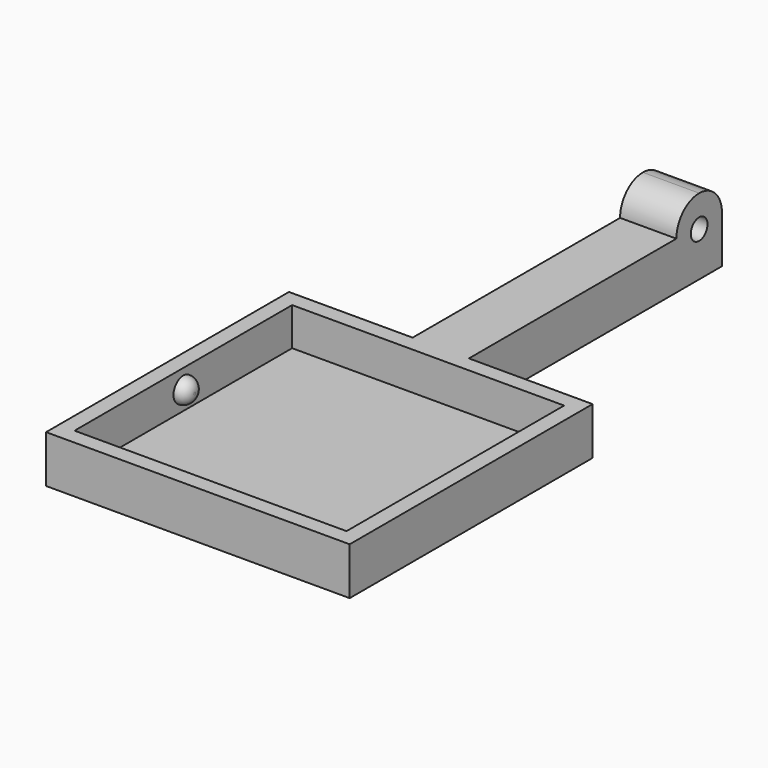
from build123d import *

# Parameters (mm, degrees)
F0_W      = 8.9
F0_H      = 50
F1_DEPTH  = 7.5
F2_W      = 43
F2_H      = 43
F3_DEPTH  = 6
F4_W      = 8.9
F4_H      = 9
F5_DEPTH  = 4.5
F6_R      = 4.49999
F7_R      = 1.95
F8_DEPTH  = 1.8
F9_R      = 1.95
F10_DEPTH = 1.8
F12_D     = 3.3
F13_R     = 1.75


# Not quite as in the source:
# - a fillet or chamfer is up to 0.001 mm smaller than in the source, because OpenCascade refuses the exact size
# - a feature names something its author has since deleted; it is built from what else it names


with BuildPart() as f1:
    # F0 (on Top) → F1 (new body)
    with BuildSketch(Plane.XY):
        Polygon((-4.45, -9.0662492651), (-24, -9.0662492651), (-24, -57.0662492651), (24, -57.0662492651), (24, -9.0662492651), (4.45, -9.0662492651), align=None)
        with Locations((0, 15.9337507349)):
            Rectangle(F0_W, F0_H)
    extrude(amount=F1_DEPTH)

    # F2 (on face) → F3 (cut)
    with BuildSketch(Plane.XY.offset(7.5)):
        with Locations((0, -33.0662492651)):
            Rectangle(F2_W, F2_H)
    extrude(amount=-F3_DEPTH, mode=Mode.SUBTRACT)

    # F4 (on face) → F5 (join)
    with BuildSketch(Plane.XY.offset(7.5)):
        with Locations((0, 36.4337507349)):
            Rectangle(F4_W, F4_H)
    extrude(amount=F5_DEPTH)

    # F6 (radius 4.5 in the source; OpenCascade refuses exactly that, so slightly less here)
    f6_edges = [f1.edges().sort_by_distance(p)[0] for p in [
        (0, 40.933751, 12),
        (0, 31.933751, 12),
    ]]
    fillet(f6_edges, radius=F6_R)

    # F7 (on face) → F8 (join)
    with BuildSketch(Plane(origin=(21.5, 0, 0), x_dir=(0, -1, 0), z_dir=(-1, 0, 0))):
        with Locations((33.0662492651, 4.5)):
            Circle(F7_R)
    extrude(amount=F8_DEPTH)

    # F9 (on face) → F10 (join)
    with BuildSketch(Plane.YZ.offset(-21.5)):
        with Locations((-33.0662492651, 4.5)):
            Circle(F9_R)
    extrude(amount=F10_DEPTH)

    # F12 (through all)
    with Locations(Plane.YZ.offset(4.45)):
        with Locations((36.4337507349, 7)):
            Hole(F12_D / 2)

    # F13
    f13_edges = [f1.edges().sort_by_distance(p)[0] for p in [
        (-19.7, -35.016249, 4.5),
        (19.7, -31.116249, 4.5),
    ]]
    fillet(f13_edges, radius=F13_R)


solid = f1.part
